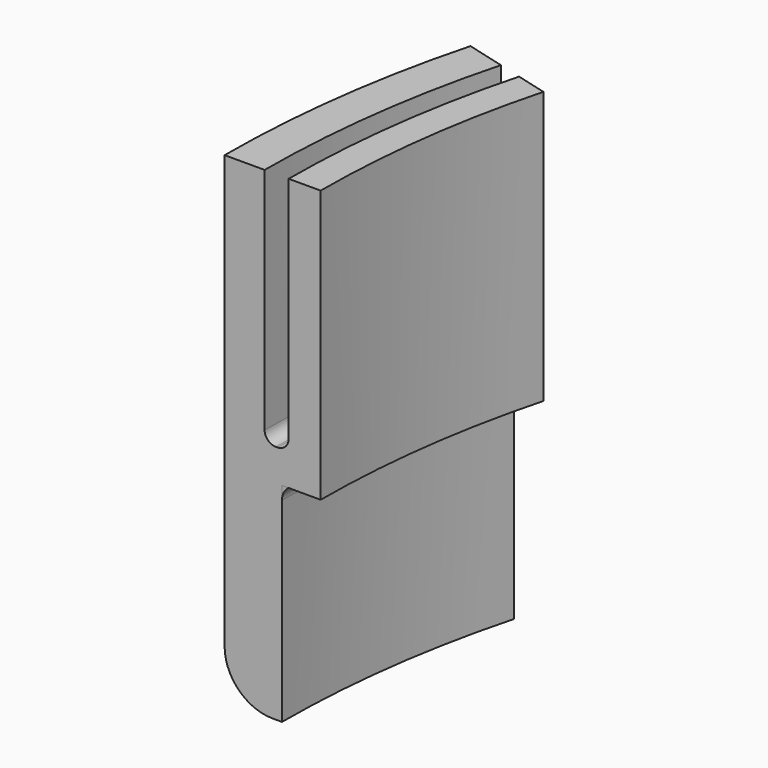
from build123d import *

# Parameters (mm, degrees)
F0_R        = 80.899
F0_R_2      = 77.724
F1_DEPTH    = 38.1
F0_R_3      = 75.819
F0_R_4      = 73.279
F2_DEPTH    = 19.05
F3_W        = 22.7063447237
F3_H        = 49.682635814
F4_ANGLE    = 15
F5_R        = 76.3482321919
F6_DEPTH    = 16.51
F7_T2_ANGLE = 15
F9_ANGLE    = 15
F10_R       = 3.81


# Not quite as in the source:
# - a fillet or chamfer that OpenCascade refuses, or shapes differently, is made with other operations: its cross-section is extruded or revolved along the edge and cut away or added


with BuildPart() as f1:
    # F0 (on Top) → F1 (new body)
    with BuildSketch(Plane.XY):
        Circle(F0_R)
        Circle(F0_R_2, mode=Mode.SUBTRACT)
    extrude(amount=F1_DEPTH)


with BuildPart() as f1b:
    # F0 (on Top) → F1, piece 2 (new body)
    with BuildSketch(Plane.XY):
        Circle(F0_R_3)
        Circle(F0_R_4, mode=Mode.SUBTRACT)
    extrude(amount=F1_DEPTH)


with BuildPart() as f2:
    # F0 (on Top) → F2 (new body)
    with BuildSketch(Plane.XY):
        Circle(F0_R_2)
        Circle(F0_R_3, mode=Mode.SUBTRACT)
    extrude(amount=F2_DEPTH)


with BuildPart() as f4_tool:
    # F3 (on Front) → F4 (revolve)
    with BuildSketch(Plane.XZ):
        with Locations((-76.5442997217, 24.841317907)):
            Rectangle(F3_W, F3_H)
    revolve(axis=Axis((0, 0, 38.7800522149), (0, 0, -1)), revolution_arc=F4_ANGLE)


with BuildPart() as f1_1:
    add(f1.part)

    # F4: intersect by f4_tool
    add(f4_tool.part, mode=Mode.INTERSECT)



with BuildPart() as f1b_1:
    add(f1b.part)

    # F4: intersect by f4_tool
    add(f4_tool.part, mode=Mode.INTERSECT)


with BuildPart() as f2_1:
    add(f2.part)

    # F4: intersect by f4_tool
    add(f4_tool.part, mode=Mode.INTERSECT)


with BuildPart() as f6_tool:
    # F5 (on Top) → F6 (new body)
    with BuildSketch(Plane.XY):
        Circle(F5_R)
    extrude(amount=F6_DEPTH)


with BuildPart() as f1b_2:
    add(f1b_1.part)

    # F6: cut by f6_tool
    add(f6_tool.part, mode=Mode.SUBTRACT)


with BuildPart() as f2_2:
    add(f2_1.part)

    # F6: cut by f6_tool
    add(f6_tool.part, mode=Mode.SUBTRACT)

    # F7: fillet of radius 1.27 on 1 edges, made by hand

    # F7_s1 → F7_t2 (revolve)
    with BuildSketch(Plane(origin=(0, 0, 0), x_dir=(0, 0, 1), z_dir=(0.2588190451, 0.9659258263, 0))):
        with BuildLine():
            ThreePointArc((15.4784172091, -76.3482321919), (16.0581261377, -76.2082045624), (16.51, -75.819))
            Line((16.51, -75.819), (16.51, -76.3482321919))
            Line((16.51, -76.3482321919), (15.4784172091, -76.3482321919))
        make_face()
    revolve(axis=Axis((0, 0, 16.51), (0, 0, 1)), revolution_arc=F7_T2_ANGLE)


with BuildPart() as f1_2:
    add(f1_1.part)

    add(f1b_2.part)  # F9 merges F1b

    add(f2_2.part)  # F9 merges F2
    # F8 (on Front) → F9 (revolve)
    with BuildSketch(Plane.XZ):
        with BuildLine():
            ThreePointArc((-75.819, 19.939), (-76.0793820715, 19.3103820715), (-76.708, 19.05))
            Line((-76.708, 19.05), (-75.819, 19.05))
            Line((-75.819, 19.05), (-75.819, 19.939))
        make_face()
        with BuildLine():
            ThreePointArc((-76.835, 19.05), (-77.4636179285, 19.3103820715), (-77.724, 19.939))
            Line((-77.724, 19.939), (-77.724, 19.05))
            Line((-77.724, 19.05), (-76.835, 19.05))
        make_face()
    revolve(axis=Axis((0, 0, 38.7800522149), (0, 0, -1)), revolution_arc=F9_ANGLE)

    # F10
    f10_edges = [f1_2.edges().sort_by_distance(p)[0] for p in [
        (-80.206898, 10.559438, 0),
    ]]
    fillet(f10_edges, radius=F10_R)


solid = f1_2.part
